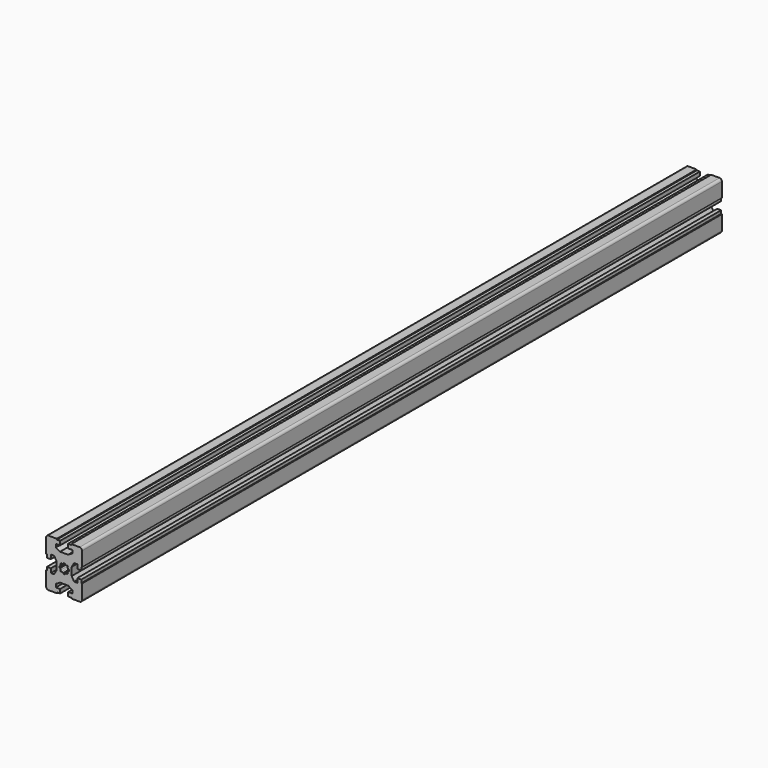
from build123d import *

# Parameters (mm, degrees)
F0_W             = 45
F0_H             = 60
F1_DEPTH         = 1000
F2_R             = 3
F3_R             = 5
F4_DEPTH         = 1000.001
F6_DEPTH         = 1000.001
F8_DEPTH         = 1000.001
F10_DEPTH        = 1000.001
F10_COPIES_COUNT = 8


# Not quite as in the source:
# - a pattern or mirror of a feature is missing from the dataset's text; its kind, count and spacing are read off the source's solid


with BuildPart() as f1:
    # F0 (on Front) → F1 (new body)
    with BuildSketch(Plane.XZ):
        Rectangle(F0_W, F0_H)
    extrude(amount=F1_DEPTH)

    # F2
    f2_edges = [f1.edges().sort_by_distance(p)[0] for p in [
        (-22.5, -500, -30),
        (-22.5, -500, 30),
        (22.5, -500, -30),
        (22.5, -500, 30),
    ]]
    fillet(f2_edges, radius=F2_R)

    # F3 (on Front) → F4 (cut, through all)
    with BuildSketch(Plane.XZ):
        Circle(F3_R)
    extrude(amount=F4_DEPTH, mode=Mode.SUBTRACT)

    # F5 (on Front) → F6 (cut, through all)
    with BuildSketch(Plane.XZ):
        Polygon((9, 30), (-9, 30), (-9, 29), (-5, 29), (-5, 24), (-10.25, 24), (-10.25, 20), (-5.0538475773, 17), (5.0538475773, 17), (10.25, 20), (10.25, 24), (5, 24), (5, 29), (9, 29), align=None)
    f6 = extrude(amount=F6_DEPTH, mode=Mode.SUBTRACT)

    # F6_copies: F6 across plane
    add(f6.mirror(Plane(origin=(0, 0, 0), x_dir=(-1, 0, 0), z_dir=(0, 0, -1))), mode=Mode.SUBTRACT)

    # F7 (on Front) → F8 (cut, through all)
    with BuildSketch(Plane.XZ):
        Polygon((-21.5, 9), (-22.5, 9), (-22.5, -9), (-21.5, -9), (-21.5, -5), (-16.5, -5), (-16.5, -10.25), (-12.5, -10.25), (-9.5, -5.0538475773), (-9.5, 5.0538475773), (-12.5, 10.25), (-16.5, 10.25), (-16.5, 5), (-21.5, 5), align=None)
    f8 = extrude(amount=F8_DEPTH, mode=Mode.SUBTRACT)

    # F8_copies: F8 across plane
    add(f8.mirror(Plane(origin=(0, 0, 0), x_dir=(0, 0, 1), z_dir=(1, 0, 0))), mode=Mode.SUBTRACT)

    # F9 (on Front) → F10 (cut, through all)
    with BuildSketch(Plane.XZ):
        with BuildLine():
            Line((0, 0), (1.041889066, 5.9088465181))
            ThreePointArc((1.041889066, 5.9088465181), (0, 6), (-1.041889066, 5.9088465181))
            Line((-1.041889066, 5.9088465181), (0, 0))
        make_face()
    f10 = extrude(amount=F10_DEPTH, mode=Mode.SUBTRACT)

    # F10_copies: F10 ×8 about axis
    f10_copies_axis = Axis((0, 0, 0), (0, 1, 0))
    for i in range(1, F10_COPIES_COUNT):
        add(f10.rotate(f10_copies_axis, i * 360 / F10_COPIES_COUNT), mode=Mode.SUBTRACT)


solid = f1.part
